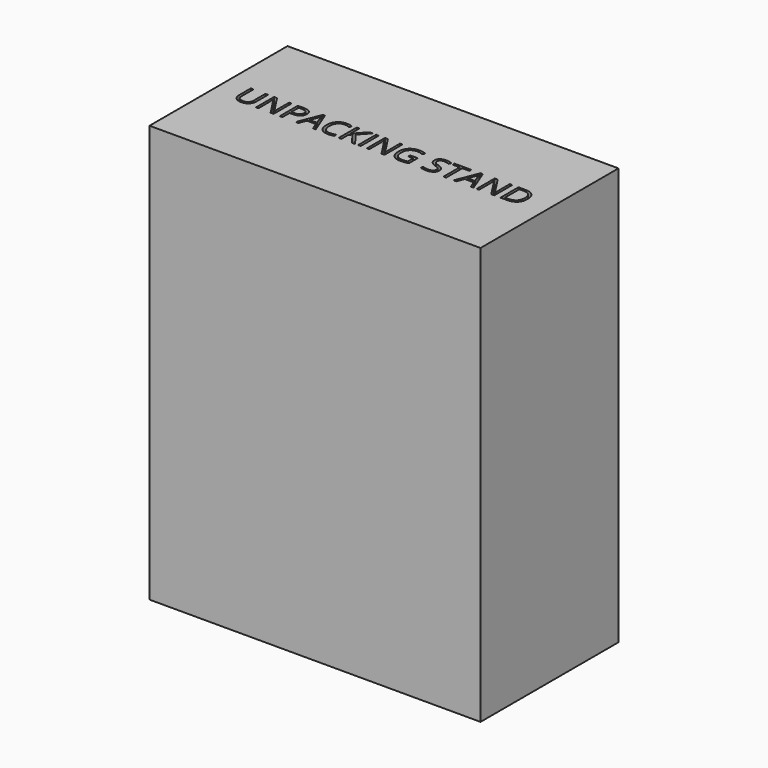
from build123d import *

# Parameters (mm, degrees)
F0_W         = 1190
F0_H         = 620
F1_DEPTH     = 1500
F2_TEXT_SIZE = 113.5087398104
F3_DEPTH     = 94


# Not quite as in the source:
# - Text() gives the source's letters only with a copy of the font that has no kerning and outlines rounded to 1/6400 em; it was checked with that copy


with BuildPart() as f1:
    # F0 (on Top) → F1 (new body)
    with BuildSketch(Plane.XY):
        Rectangle(F0_W, F0_H)
    extrude(amount=F1_DEPTH)

    # F2 (on face) → F3 (cut)
    with BuildSketch(Plane.XY.offset(1500)):
        with Locations((-525, -36.134259519)):
            Text('UNPACKING STAND', F2_TEXT_SIZE, font='Open Sans', text_align=(TextAlign.LEFT, TextAlign.BOTTOM))
    extrude(amount=-F3_DEPTH, mode=Mode.SUBTRACT)


solid = f1.part
